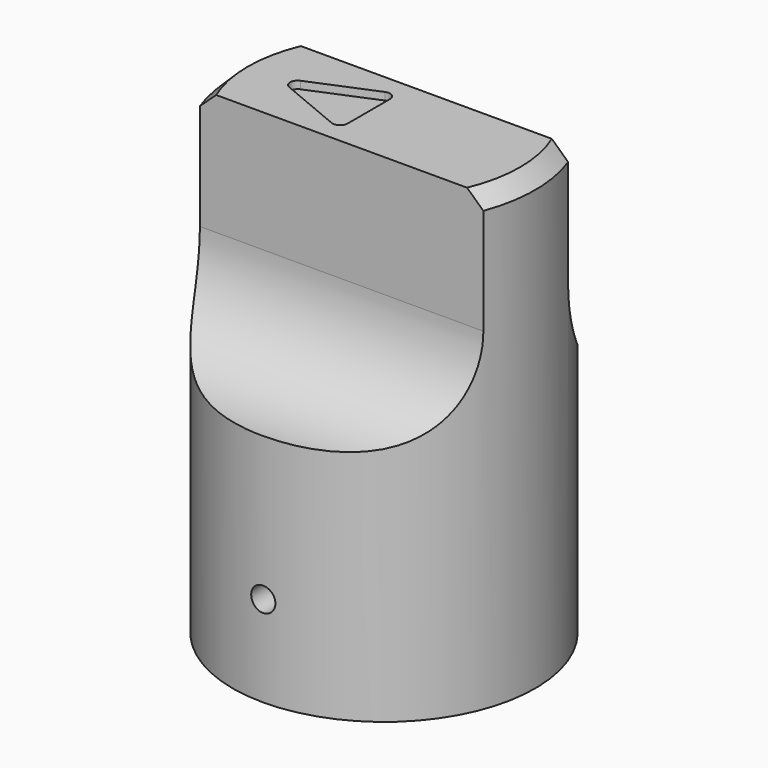
from build123d import *

# Parameters (mm, degrees)
F3_DEPTH  = 12.5
F4_SIZE   = 1
F6_DEPTH  = 14.5
F7_R      = 0.5
F8_R      = 0.8
F9_DEPTH  = 12.5
F10_SIZE  = 1
F12_DEPTH = 0.5
F13_R     = 0.5


# Not quite as in the source:
# - a pattern or mirror of a feature is missing from the dataset's text; its kind, count and spacing are read off the source's solid


with BuildPart() as f1:
    # F0 (on Right) → F1 (revolve)
    with BuildSketch(Plane.YZ):
        Polygon((-10, 0), (-8, 0), (-8, 14.5), (0, 14.5), (0, 30), (-10, 30), align=None)
    revolve(axis=Axis((0, 0, 22.25), (0, 0, 1)))

    # F2 (on Right) → F3 (cut, symmetric)
    with BuildSketch(Plane.YZ):
        with BuildLine():
            Line((-3.5, 22), (-3.5, 30))
            Line((-3.5, 30), (-10, 30))
            Line((-10, 30), (-10, 15.5))
            ThreePointArc((-10, 15.5), (-5.4038059223, 17.4038059223), (-3.5, 22))
        make_face()
    f3 = extrude(amount=F3_DEPTH, both=True, mode=Mode.SUBTRACT)

    # F3_copies: F3 across plane
    add(f3.mirror(Plane.ZX.offset(1e-06)), mode=Mode.SUBTRACT)

    # F4
    f4_edges = [f1.edges().sort_by_distance(p)[0] for p in [
        (10, 1e-06, 30),
    ]]
    chamfer(f4_edges, length=F4_SIZE)

    # F5 (on face) → F6 (join, through all)
    with BuildSketch(Plane(origin=(0, 0, 0), x_dir=(1, 0, 0), z_dir=(0, 0, -1))):
        with BuildLine():
            ThreePointArc((-7.3653645844, 3.1227238973), (-8, 0), (-7.3653645844, -3.1227238973))
            ThreePointArc((-7.3653645844, -3.1227238973), (-5.2, 0), (-7.3653645844, 3.1227238973))
        make_face()
        with BuildLine():
            ThreePointArc((3.1227238973, 7.3653645844), (0, 8), (-3.1227238973, 7.3653645844))
            ThreePointArc((-3.1227238973, 7.3653645844), (0, 5.2), (3.1227238973, 7.3653645844))
        make_face()
        with BuildLine():
            ThreePointArc((7.3653645844, -3.1227238973), (8, 0), (7.3653645844, 3.1227238973))
            ThreePointArc((7.3653645844, 3.1227238973), (5.2, 0), (7.3653645844, -3.1227238973))
        make_face()
        with BuildLine():
            ThreePointArc((-3.1227238973, -7.3653645844), (0, -8), (3.1227238973, -7.3653645844))
            ThreePointArc((3.1227238973, -7.3653645844), (0, -5.2), (-3.1227238973, -7.3653645844))
        make_face()
    extrude(amount=-F6_DEPTH)

    # F7
    f7_edges = [f1.edges().sort_by_distance(p)[0] for p in [
        (3.122724, -7.365365, 7.25),
        (-7.365365, 3.122724, 7.25),
        (-7.365365, -3.122724, 7.25),
        (3.122724, 7.365365, 7.25),
        (-3.122724, 7.365365, 7.25),
        (7.365365, 3.122724, 7.25),
        (7.365365, -3.122724, 7.25),
        (-3.122724, -7.365365, 7.25),
    ]]
    fillet(f7_edges, radius=F7_R)

    # F8 (on Front) → F9 (cut, symmetric)
    with BuildSketch(Plane.XZ):
        with Locations((0, 6)):
            Circle(F8_R)
    extrude(amount=F9_DEPTH, both=True, mode=Mode.SUBTRACT)

    # F10
    f10_edges = [f1.edges().sort_by_distance(p)[0] for p in [
        (-5.656854, 5.656854, 0),
        (5.656854, -5.656854, 0),
        (3.218481, -7.178495, 0),
        (7.178495, -3.218481, 0),
        (0, -5.2, 0),
        (5.2, 0, 0),
        (-3.218481, -7.178495, 0),
        (7.178495, 3.218481, 0),
        (-5.656854, -5.656854, 0),
        (5.656854, 5.656854, 0),
        (-7.178495, -3.218481, 0),
        (3.218481, 7.178495, 0),
        (-5.2, 0, 0),
        (0, 5.2, 0),
        (-7.178495, 3.218481, 0),
        (-3.218481, 7.178495, 0),
        (-10, 1e-06, 30),
    ]]
    chamfer(f10_edges, length=F10_SIZE)

    # F11 (on face) → F12 (cut)
    with BuildSketch(Plane.XY.offset(30)):
        Polygon((-1, 2.5), (-7, 0), (-1, -2.5), align=None)
    extrude(amount=-F12_DEPTH, mode=Mode.SUBTRACT)

    # F13
    f13_edges = [f1.edges().sort_by_distance(p)[0] for p in [
        (-1, 2.5, 29.75),
        (-1, -2.5, 29.75),
        (-7, 0, 29.75),
    ]]
    fillet(f13_edges, radius=F13_R)


solid = f1.part
